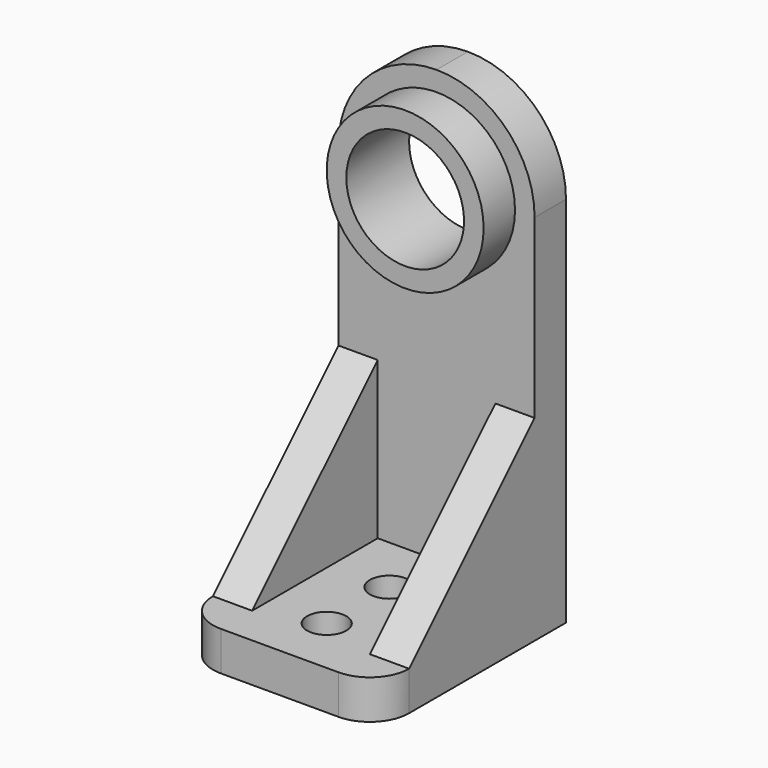
from build123d import *

# Parameters (mm, degrees)
F1_DEPTH = 25
F3_DEPTH = 10
F4_R     = 20
F5_DEPTH = 10
F6_R     = 24.99999
F8_D     = 30
F9_R     = 10
F11_D    = 10


# Not quite as in the source:
# - a fillet or chamfer is up to 0.001 mm smaller than in the source, because OpenCascade refuses the exact size
# - a pattern or mirror of a feature is missing from the dataset's text; its kind, count and spacing are read off the source's solid


with BuildPart() as f1:
    # F0 (on Right) → F1 (new body, symmetric)
    with BuildSketch(Plane.YZ):
        Polygon((-60, 0), (0, 0), (0, 120), (-10, 120), (-10, 10), (-60, 10), align=None)
    extrude(amount=F1_DEPTH, both=True)

    # F2 (on face) → F3 (join)
    with BuildSketch(Plane.YZ.offset(25)):
        Polygon((-50, 10), (-10, 10), (-10, 50), align=None)
    f3 = extrude(amount=-F3_DEPTH)

    # F3_copies: F3 across plane
    add(f3.mirror(Plane(origin=(0, 0, 0), x_dir=(0, 0, -1), z_dir=(-1, 0, 0))))

    # F4 (on face) → F5 (join)
    with BuildSketch(Plane.XZ.offset(10)):
        with Locations((0, 95)):
            Circle(F4_R)
    extrude(amount=F5_DEPTH)

    # F6 (radius 25 in the source; OpenCascade refuses exactly that, so slightly less here)
    f6_edges = [f1.edges().sort_by_distance(p)[0] for p in [
        (-25, -5, 120),
        (25, -5, 120),
    ]]
    fillet(f6_edges, radius=F6_R)

    # F8 (through all)
    with Locations(Plane.XZ.offset(20)):
        with Locations((0, 95)):
            Hole(F8_D / 2)

    # F9
    f9_edges = [f1.edges().sort_by_distance(p)[0] for p in [
        (-25, -60, 5),
        (25, -60, 5),
    ]]
    fillet(f9_edges, radius=F9_R)

    # F11 (through all)
    with Locations(Plane.XY.offset(10)):
        with Locations((0, -25), (0, -45)):
            Hole(F11_D / 2)


solid = f1.part
